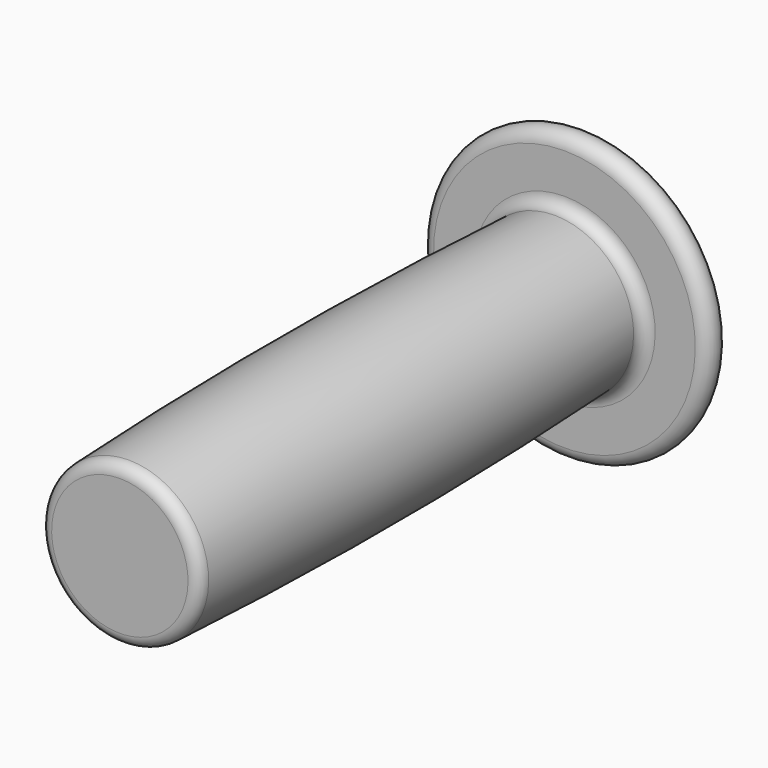
from build123d import *


# Not quite as in the source:
# - a feature names something its author has since deleted; it is built from what else it names


with BuildPart() as f1:
    # F0 (on Right) → F1 (revolve)
    with BuildSketch(Plane.YZ):
        with BuildLine():
            Line((-4.49999996, 22.3697591573), (-4.49999996, 15.5121270956))
            ThreePointArc((-4.49999996, 15.5121270956), (-5.128710844, 14.0562541066), (-6.6195661202, 13.5157043114))
            ThreePointArc((-6.6195661202, 13.5157043114), (-52.1013620917, 14.6000076136), (-97.5862327976, 13.6534267626))
            ThreePointArc((-97.5862327976, 13.6534267626), (-98.9443797276, 13.038676402), (-99.5, 11.6552866512))
            Line((-99.5, 11.6552866512), (-99.5, 0))
            Line((-99.5, 0), (-38.1620294721, 0))
            ThreePointArc((-38.1620294721, 0), (-37.1369032063, 2.4748737342), (-34.6620294721, 3.5))
            Line((-34.6620294721, 3.5), (0, 3.5))
            Line((0, 3.5), (0, 22.3697591573))
            ThreePointArc((0, 22.3697591573), (-2.24999998, 24.5060521618), (-4.49999996, 22.3697591573))
        make_face()
    revolve(axis=Axis((0, -59.5094561577, 0), (0, -1, 0)))


solid = f1.part
